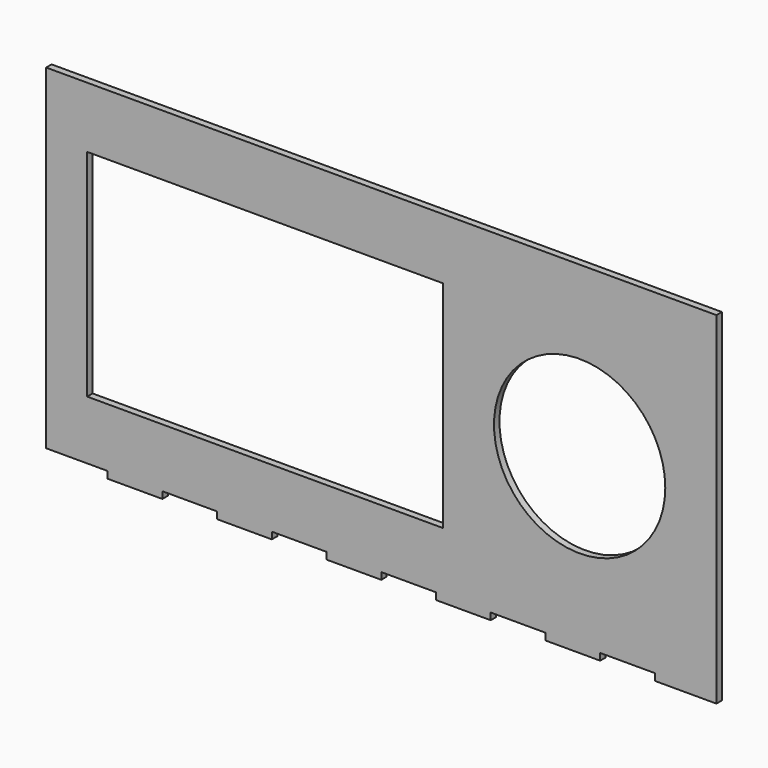
from build123d import *

# Parameters (mm, degrees)
F1_DEPTH = 3.175
F2_W     = 165.1
F2_H     = 100
F2_R     = 39.75
F3_DEPTH = 25.4
F4_W     = 3.175
F4_H     = 25.4
F4_H_2   = 28.575
F4_W_2   = 25.4
F4_H_3   = 3.175
F5_DEPTH = 3.175


# Not quite as in the source:
# - a length typed as a fraction of an inch, garbled in the dataset ("3 / 203.2 mm" for 3/8 in), is restored


with BuildPart() as f1:
    # F0 (on Front) → F1 (new body)
    with BuildSketch(Plane.XZ):
        Polygon((-178.9622853069, -44.2643848114), (-153.5622853069, -44.2643848114), (-153.5622853069, -47.4393848114), (-128.1622853069, -47.4393848114), (-128.1622853069, -44.2643848114), (-102.7622853069, -44.2643848114), (-102.7622853069, -47.4393848114), (-77.3622853069, -47.4393848114), (-77.3622853069, -44.2643848114), (-51.9622853069, -44.2643848114), (-51.9622853069, -47.4393848114), (-26.5622853069, -47.4393848114), (-26.5622853069, -44.2643848114), (-1.1622853069, -44.2643848114), (-1.1622853069, -47.4393848114), (24.2377146931, -47.4393848114), (24.2377146931, -44.2643848114), (49.6377146931, -44.2643848114), (49.6377146931, -47.4393848114), (75.0377146931, -47.4393848114), (75.0377146931, -44.2643848114), (100.4377146931, -44.2643848114), (100.4377146931, -47.4393848114), (125.8377146931, -47.4393848114), (129.0127146931, -47.4393848114), (129.0127146931, -44.2643848114), (129.0127146931, -18.8643848114), (125.8377146931, -18.8643848114), (125.8377146931, 6.5356151886), (129.0127146931, 6.5356151886), (129.0127146931, 31.9356151886), (125.8377146931, 31.9356151886), (125.8377146931, 57.3356151886), (129.0127146931, 57.3356151886), (129.0127146931, 82.7356151886), (125.8377146931, 82.7356151886), (125.8377146931, 108.1356151886), (125.8377146931, 111.3106151886), (100.4377146931, 111.3106151886), (100.4377146931, 108.1356151886), (75.0377146931, 108.1356151886), (75.0377146931, 111.3106151886), (49.6377146931, 111.3106151886), (49.6377146931, 108.1356151886), (24.2377146931, 108.1356151886), (24.2377146931, 111.3106151886), (-1.1622853069, 111.3106151886), (-1.1622853069, 108.1356151886), (-26.5622853069, 108.1356151886), (-26.5622853069, 111.3106151886), (-51.9622853069, 111.3106151886), (-51.9622853069, 108.1356151886), (-77.3622853069, 108.1356151886), (-77.3622853069, 111.3106151886), (-102.7622853069, 111.3106151886), (-102.7622853069, 108.1356151886), (-128.1622853069, 108.1356151886), (-128.1622853069, 111.3106151886), (-153.5622853069, 111.3106151886), (-153.5622853069, 108.1356151886), (-178.9622853069, 108.1356151886), (-178.9622853069, 82.7356151886), (-182.1372853069, 82.7356151886), (-182.1372853069, 57.3356151886), (-178.9622853069, 57.3356151886), (-178.9622853069, 31.9356151886), (-182.1372853069, 31.9356151886), (-182.1372853069, 6.5356151886), (-178.9622853069, 6.5356151886), (-178.9622853069, -18.8643848114), (-182.1372853069, -18.8643848114), (-182.1372853069, -44.2643848114), align=None)
    extrude(amount=F1_DEPTH)

    # F2 (on face) → F3 (cut)
    with BuildSketch(Plane.XZ.offset(3.175)):
        with Locations((-80.5372853069, 33.0406151886)):
            Rectangle(F2_W, F2_H)
        with Locations((65.5127146931, 33.0406151886)):
            Circle(F2_R)
    extrude(amount=-F3_DEPTH, mode=Mode.SUBTRACT)

    # F4 (on face) → F5 (join)
    with BuildSketch(Plane.XZ.offset(3.175)):
        Polygon((-182.1372853069, 111.3106151886), (-182.1372853069, 82.7356151886), (-178.9622853069, 82.7356151886), (-178.9622853069, 108.1356151886), (-153.5622853069, 108.1356151886), (-153.5622853069, 111.3106151886), align=None)
        with Locations((-180.5497853069, 44.6356151886)):
            Rectangle(F4_W, F4_H)
        with Locations((-180.5497853069, -6.1643848114)):
            Rectangle(F4_W, F4_H)
        with Locations((127.4252146931, -6.1643848114)):
            Rectangle(F4_W, F4_H)
        with Locations((127.4252146931, 44.6356151886)):
            Rectangle(F4_W, F4_H)
        with Locations((127.4252146931, 97.0231151886)):
            Rectangle(F4_W, F4_H_2)
        with Locations((87.7377146931, 109.7231151886)):
            Rectangle(F4_W_2, F4_H_3)
        with Locations((36.9377146931, 109.7231151886)):
            Rectangle(F4_W_2, F4_H_3)
        with Locations((-13.8622853069, 109.7231151886)):
            Rectangle(F4_W_2, F4_H_3)
        with Locations((-64.6622853069, 109.7231151886)):
            Rectangle(F4_W_2, F4_H_3)
        with Locations((-115.4622853069, 109.7231151886)):
            Rectangle(F4_W_2, F4_H_3)
    extrude(amount=-F5_DEPTH)


solid = f1.part
